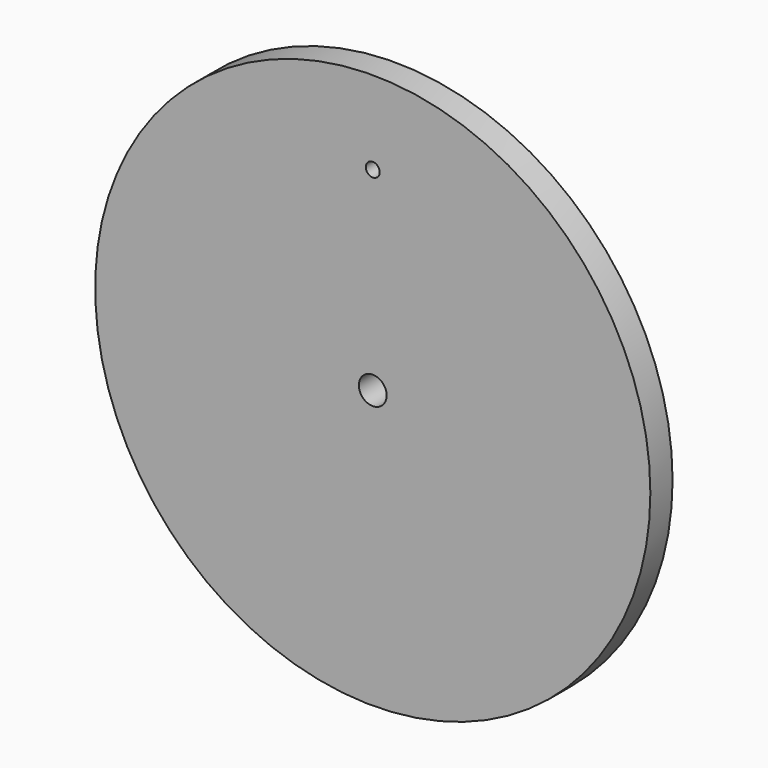
from build123d import *

# Parameters (mm, degrees)
F0_R     = 63.5
F0_R_2   = 3.175
F0_R_3   = 1.5875
F1_DEPTH = 6.35


# Not quite as in the source:
# - a length typed as a fraction of an inch, garbled in the dataset ("3 / 203.2 mm" for 3/8 in), is restored


with BuildPart() as f1:
    # F0 (on Front) → F1 (new body)
    with BuildSketch(Plane.XZ):
        Circle(F0_R)
        Circle(F0_R_2, mode=Mode.SUBTRACT)
        with Locations((0, 44.45)):
            Circle(F0_R_3, mode=Mode.SUBTRACT)
    extrude(amount=F1_DEPTH)


solid = f1.part
